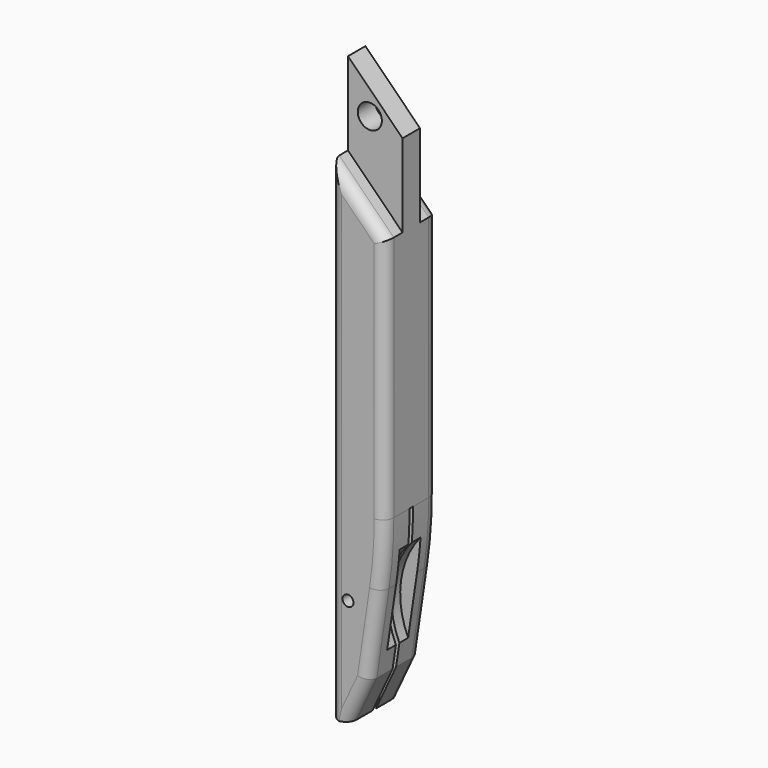
from build123d import *

# Parameters (mm, degrees)
F0_R          = 25
F1_DEPTH      = 150
F0_R_2        = 55.1997583715
F2_DEPTH      = 50
F4_DEPTH      = 250.001
F8_DEPTH      = 60
F10_R         = 40
F11_DEPTH     = 257
F12_T1_DEPTH  = 1255
F12_T3_DEPTH  = 2500
F12_T5_DEPTH  = 603.5533905933
F12_T7_DEPTH  = 556.1937137964
F12_T9_DEPTH  = 595.9370668734
F12_T14_DEPTH = 330
F12_S15_R     = 50
F12_T16_DEPTH = 170
F12_T20_DEPTH = 330
F12_S21_R     = 50
F12_T22_DEPTH = 170
F12_T26_DEPTH = 330
F12_S27_R     = 50
F12_T28_DEPTH = 170
F12_T32_DEPTH = 330
F12_S33_R     = 50
F12_T34_DEPTH = 170
F12_T36_ANGLE = 8.4091330213
F12_T38_ANGLE = 8.4091330213


# Not quite as in the source:
# - a fillet or chamfer that OpenCascade refuses, or shapes differently, is made with other operations: its cross-section is extruded or revolved along the edge and cut away or added


with BuildPart() as f1:
    # F0 (on Front) → F1 (new body)
    with BuildSketch(Plane.XZ):
        with BuildLine():
            Line((250, 824.2658257814), (0, 1074.2658257814))
            Line((0, 1074.2658257814), (0, -1175.7341742186))
            Line((0, -1175.7341742186), (80, -1175.7341742186))
            Line((80, -1175.7341742186), (172.4239571783, -977.530358429))
            Line((172.4239571783, -977.530358429), (228.4980691431, -598.2156102055))
            ThreePointArc((228.4980691431, -598.2156102055), (244.6172738506, -452.3695412242), (250, -305.7341742186))
            Line((250, -305.7341742186), (250, 824.2658257814))
        make_face()
        with Locations((80, -675.7341742186)):
            Circle(F0_R, mode=Mode.SUBTRACT)
    extrude(amount=F1_DEPTH)

    # F0 (on Front) → F2 (join)
    with BuildSketch(Plane.XZ):
        Polygon((0, 1454.2658257814), (0, 1074.2658257814), (250, 824.2658257814), (250, 1204.2658257814), align=None)
        with Locations((100, 1244.2658257814)):
            Circle(F0_R_2, mode=Mode.SUBTRACT)
    extrude(amount=F2_DEPTH)

    # F3 (on face) → F4 (cut, through all)
    with BuildSketch(Plane(origin=(0, 0, 0), x_dir=(0, -1, 0), z_dir=(-1, 0, 0))):
        Polygon((10, -1175.7341742186), (10, -305.7341742186), (0, -305.7341742186), (0, -598.2156102055), (0, -977.530358429), (0, -1175.7341742186), align=None)
    extrude(amount=-F4_DEPTH, mode=Mode.SUBTRACT)

    # F5: F1 across plane


with BuildPart() as f1_1:
    add(f1.part)
    add(f1.part.mirror(Plane.XZ))

    # F7 (on offset) → F8 (cut, symmetric)
    with BuildSketch(Plane(origin=(0, 0, 0), x_dir=(-1, 0, 0), z_dir=(0, 1, 0))):
        with BuildLine():
            Line((-228.4980691431, -598.2156102055), (-187.4724905077, -875.7341742186))
            ThreePointArc((-187.4724905077, -875.7341742186), (-154.7929091893, -655.7842074431), (-244.6172738506, -452.3695412242))
            Line((-244.6172738506, -452.3695412242), (-228.4980691431, -598.2156102055))
        make_face()
        Polygon((-289.7645564147, -893.9040561501), (-187.4724905077, -875.7341742186), (-228.4980691431, -598.2156102055), (-244.6172738506, -452.3695412242), (-337.4301303856, -462.6274072361), align=None)
    extrude(amount=F8_DEPTH, both=True, mode=Mode.SUBTRACT)

    # F10 (on face) → F11 (cut)
    with BuildSketch(Plane(origin=(-313.6375788675, 0, -1085.0784920755), x_dir=(0.9606739331, 0, -0.2776789409), z_dir=(-0.2776789409, 0, -0.9606739331))):
        with Locations((364.9035775946, 0)):
            Circle(F10_R)
    extrude(amount=-F11_DEPTH, mode=Mode.SUBTRACT)

    # F12: fillet of radius 50 on 14 edges, made by hand

    # F12_s2 → F12_t1 (cut)
    with BuildSketch(Plane.XY.offset(-305.7341742186)):
        with BuildLine():
            ThreePointArc((250, -100), (235.3553390593, -135.3553390593), (200, -150))
            Line((200, -150), (250, -150))
            Line((250, -150), (250, -100))
        make_face()
        with BuildLine():
            ThreePointArc((250, 100), (235.3553390593, 135.3553390593), (200, 150))
            Line((200, 150), (250, 150))
            Line((250, 150), (250, 100))
        make_face()
    extrude(amount=F12_T1_DEPTH, mode=Mode.SUBTRACT)

    # F12_s4 → F12_t3 (cut)
    with BuildSketch(Plane.XY.offset(-1300.7341742186)):
        with BuildLine():
            ThreePointArc((50, -150), (14.6446609407, -135.3553390593), (0, -100))
            Line((0, -100), (0, -150))
            Line((0, -150), (50, -150))
        make_face()
        with BuildLine():
            ThreePointArc((50, 150), (14.6446609407, 135.3553390593), (0, 100))
            Line((0, 100), (0, 150))
            Line((0, 150), (50, 150))
        make_face()
    extrude(amount=F12_T3_DEPTH, mode=Mode.SUBTRACT)

    # F12_s6 → F12_t5 (cut)
    with BuildSketch(Plane(origin=(-198.7445652424, 0, 198.7445652424), x_dir=(0, 1, 0), z_dir=(-0.7071067812, 0, 0.7071067812))):
        with BuildLine():
            ThreePointArc((-150, -709.620650207), (-135.3553390593, -744.9759892663), (-100, -759.620650207))
            Line((-100, -759.620650207), (-150, -759.620650207))
            Line((-150, -759.620650207), (-150, -709.620650207))
        make_face()
        with BuildLine():
            ThreePointArc((100, -759.620650207), (135.3553390593, -744.9759892663), (150, -709.620650207))
            Line((150, -709.620650207), (150, -759.620650207))
            Line((150, -759.620650207), (100, -759.620650207))
        make_face()
    extrude(amount=F12_T5_DEPTH, mode=Mode.SUBTRACT)

    # F12_s8 → F12_t7 (cut)
    with BuildSketch(Plane(origin=(-488.8711024777, 0, -1048.3874625005), x_dir=(0, 1, 0), z_dir=(0.4226182617, 0, 0.906307787))):
        with BuildLine():
            ThreePointArc((-150, -519.3913559403), (-135.3553390593, -554.7466949997), (-100, -569.3913559403))
            Line((-100, -569.3913559403), (-150, -569.3913559403))
            Line((-150, -569.3913559403), (-150, -519.3913559403))
        make_face()
        with BuildLine():
            ThreePointArc((150, -519.3913559403), (135.3553390593, -554.7466949997), (100, -569.3913559403))
            Line((100, -569.3913559403), (150, -569.3913559403))
            Line((150, -569.3913559403), (150, -519.3913559403))
        make_face()
    extrude(amount=F12_T7_DEPTH, mode=Mode.SUBTRACT)

    # F12_s10 → F12_t9 (cut)
    with BuildSketch(Plane(origin=(-168.8064738845, 0, -1141.8956608733), x_dir=(0, 1, 0), z_dir=(0.146240718, 0, 0.9892490346))):
        with BuildLine():
            ThreePointArc((-150, -263.5249746526), (-135.3553390593, -298.8803137119), (-100, -313.5249746526))
            Line((-100, -313.5249746526), (-150, -313.5249746526))
            Line((-150, -313.5249746526), (-150, -263.5249746526))
        make_face()
        with BuildLine():
            ThreePointArc((150, -263.5249746526), (135.3553390593, -298.8803137119), (100, -313.5249746526))
            Line((100, -313.5249746526), (150, -313.5249746526))
            Line((150, -313.5249746526), (150, -263.5249746526))
        make_face()
    extrude(amount=F12_T9_DEPTH, mode=Mode.SUBTRACT)


with BuildPart() as f12_tool12:
    # F12_s13 → F12_t14 (new body)
    with BuildSketch(Plane.YZ.offset(-125)):
        with BuildLine():
            ThreePointArc((-150, -1125.7341742186), (-135.3553390593, -1161.0895132779), (-100, -1175.7341742186))
            Line((-100, -1175.7341742186), (-150, -1175.7341742186))
            Line((-150, -1175.7341742186), (-150, -1125.7341742186))
        make_face()
    extrude(amount=F12_T14_DEPTH)

    # F12_s15 → F12_t16 (cut, symmetric)
    with BuildSketch(Plane(origin=(-433.606336546, 0, -929.8717894996), x_dir=(0, 1, 0), z_dir=(-0.4226182617, 0, -0.906307787))):
        with Locations((-100, 519.3913559403)):
            Circle(F12_S15_R)
    extrude(amount=F12_T16_DEPTH, both=True, mode=Mode.SUBTRACT)


with BuildPart() as f1_2:
    add(f1_1.part)

    # F12_t11: cut F12_tool12
    add(f12_tool12.part, mode=Mode.SUBTRACT)


with BuildPart() as f12_tool18:
    # F12_s19 → F12_t20 (new body)
    with BuildSketch(Plane.YZ.offset(-125)):
        with BuildLine():
            ThreePointArc((-150, -1125.7341742186), (-135.3553390593, -1161.0895132779), (-100, -1175.7341742186))
            Line((-100, -1175.7341742186), (-150, -1175.7341742186))
            Line((-150, -1175.7341742186), (-150, -1125.7341742186))
        make_face()
    extrude(amount=F12_T20_DEPTH)

    # F12_s21 → F12_t22 (cut, symmetric)
    with BuildSketch(Plane.XY.offset(-1150.7)):
        with Locations((50, -100)):
            Circle(F12_S21_R)
    extrude(amount=F12_T22_DEPTH, both=True, mode=Mode.SUBTRACT)


with BuildPart() as f1_3:
    add(f1_2.part)

    # F12_t17: cut F12_tool18
    add(f12_tool18.part, mode=Mode.SUBTRACT)


with BuildPart() as f12_tool24:
    # F12_s25 → F12_t26 (new body)
    with BuildSketch(Plane.YZ.offset(-125)):
        with BuildLine():
            ThreePointArc((150, -1125.7341742186), (135.3553390593, -1161.0895132779), (100, -1175.7341742186))
            Line((100, -1175.7341742186), (150, -1175.7341742186))
            Line((150, -1175.7341742186), (150, -1125.7341742186))
        make_face()
    extrude(amount=F12_T26_DEPTH)

    # F12_s27 → F12_t28 (cut, symmetric)
    with BuildSketch(Plane(origin=(-433.606336546, 0, -929.8717894996), x_dir=(0, 1, 0), z_dir=(-0.4226182617, 0, -0.906307787))):
        with Locations((100, 519.3913559403)):
            Circle(F12_S27_R)
    extrude(amount=F12_T28_DEPTH, both=True, mode=Mode.SUBTRACT)


with BuildPart() as f1_4:
    add(f1_3.part)

    # F12_t23: cut F12_tool24
    add(f12_tool24.part, mode=Mode.SUBTRACT)


with BuildPart() as f12_tool30:
    # F12_s31 → F12_t32 (new body)
    with BuildSketch(Plane.YZ.offset(-125)):
        with BuildLine():
            ThreePointArc((150, -1125.7341742186), (135.3553390593, -1161.0895132779), (100, -1175.7341742186))
            Line((100, -1175.7341742186), (150, -1175.7341742186))
            Line((150, -1175.7341742186), (150, -1125.7341742186))
        make_face()
    extrude(amount=F12_T32_DEPTH)

    # F12_s33 → F12_t34 (cut, symmetric)
    with BuildSketch(Plane.XY.offset(-1150.7)):
        with Locations((50, 100)):
            Circle(F12_S33_R)
    extrude(amount=F12_T34_DEPTH, both=True, mode=Mode.SUBTRACT)


with BuildPart() as f1_5:
    add(f1_4.part)

    # F12_t29: cut F12_tool30
    add(f12_tool30.part, mode=Mode.SUBTRACT)

    # F12_s35 → F12_t36 (revolve, cut)
    with BuildSketch(Plane(origin=(-81.6562093461, 0, -552.3654928034), x_dir=(0, 1, 0), z_dir=(-0.146240718, 0, -0.9892490346))):
        with BuildLine():
            ThreePointArc((-100, 313.5249746526), (-135.3553390593, 298.8803137119), (-150, 263.5249746526))
            Line((-150, 263.5249746526), (-150, 313.5249746526))
            Line((-150, 313.5249746526), (-100, 313.5249746526))
        make_face()
    revolve(axis=Axis((-1749.9999999999, -150, -305.7341742186), (0, -1, 0)), revolution_arc=F12_T36_ANGLE, mode=Mode.SUBTRACT)

    # F12_s37 → F12_t38 (revolve, cut)
    with BuildSketch(Plane(origin=(-81.6562093461, 0, -552.3654928034), x_dir=(0, 1, 0), z_dir=(-0.146240718, 0, -0.9892490346))):
        with BuildLine():
            ThreePointArc((150, 263.5249746526), (135.3553390593, 298.8803137119), (100, 313.5249746526))
            Line((100, 313.5249746526), (150, 313.5249746526))
            Line((150, 313.5249746526), (150, 263.5249746526))
        make_face()
    revolve(axis=Axis((-1749.9999999999, 150, -305.7341742186), (0, -1, 0)), revolution_arc=F12_T38_ANGLE, mode=Mode.SUBTRACT)


solid = f1_5.part
